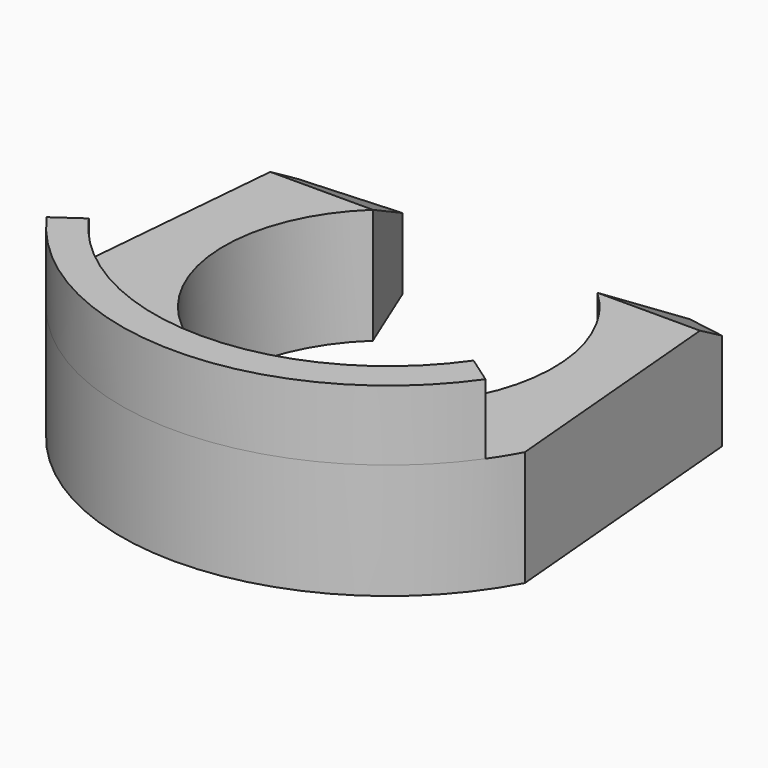
from build123d import *

# Parameters (mm, degrees)
F2_DEPTH = 2.8
F4_DEPTH = 1.7
F6_DEPTH = 12.5


# Not quite as in the source:
# - a feature of the source that left no trace in its solid (it failed there, or was rolled back) is left out


with BuildPart() as f2:
    # F1 (on Top) → F2 (new body)
    with BuildSketch(Plane.XY):
        with BuildLine():
            Line((-5.1537473182, 3.6727124144), (-5.7416372565, -3.0469003289))
            ThreePointArc((-5.7416372565, -3.0469003289), (0, -6.5), (5.7416372565, -3.0469003289))
            Line((5.7416372565, -3.0469003289), (5.1537473182, 3.6727124144))
            Line((5.1537473182, 3.6727124144), (3.4859795486, 4.7765922388))
            Line((3.4859795486, 4.7765922388), (2.7272692442, 2.9260899627))
            ThreePointArc((2.7272692442, 2.9260899627), (0, -4), (-2.7272692442, 2.9260899627))
            Line((-2.7272692442, 2.9260899627), (-3.4859795486, 4.7765922388))
            Line((-3.4859795486, 4.7765922388), (-5.1537473182, 3.6727124144))
        make_face()
    extrude(amount=F2_DEPTH)

    # F3 (on face) → F4 (join)
    with BuildSketch(Plane.XY.offset(2.8)):
        with BuildLine():
            Line((-4.6721311475, -3.2651478589), (-5.3278688525, -3.723414225))
            ThreePointArc((-5.3278688525, -3.723414225), (0, -6.5), (5.3278688525, -3.723414225))
            Line((5.3278688525, -3.723414225), (4.6721311475, -3.2651478589))
            ThreePointArc((4.6721311475, -3.2651478589), (0, -5.7), (-4.6721311475, -3.2651478589))
        make_face()
    extrude(amount=F4_DEPTH)

    # F5 (on Right) → F6 (cut, symmetric)
    with BuildSketch(Plane.YZ):
        Polygon((6.7765922388, 2.8), (2.9260899627, 2.8), (6.7765922388, 0.5769114744), align=None)
    extrude(amount=F6_DEPTH, both=True, mode=Mode.SUBTRACT)


solid = f2.part
